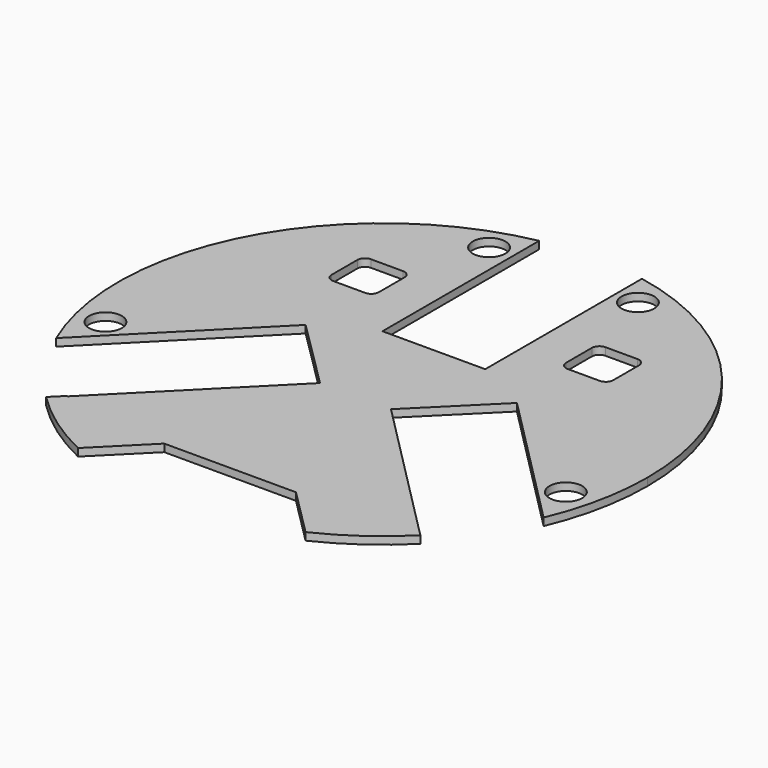
from build123d import *

# Parameters (mm, degrees)
F0_R     = 6.5
F1_DEPTH = 3


with BuildPart() as f1:
    # F0 (on Top) → F1 (new body)
    with BuildSketch(Plane.XY):
        with BuildLine():
            Line((-69.5263431778, -69.5263431778), (-74.2462120246, -74.2462120246))
            ThreePointArc((-74.2462120246, -74.2462120246), (-60.5690845883, -85.7693767736), (-45.1347826829, -94.804279398))
            Line((-45.1347826829, -94.804279398), (-26.1228149757, -75.7923116907))
            Line((-26.1228149757, -75.7923116907), (0, -49.6694967151))
            Line((0, -49.6694967151), (0, 0))
            Line((0, 0), (-13.8767590343, -13.8767590343))
            Line((-13.8767590343, -13.8767590343), (-13.825551364, -13.9276425795))
            Line((-13.825551364, -13.9276425795), (-69.2978968304, -69.7533435465))
            Line((-69.2978968304, -69.7533435465), (-69.5263431778, -69.5263431778))
        make_face()
        Polygon((0, -49.6694967151), (-26.1228149757, -75.7923116907), (0, -75.7923116907), (0, -64.7160249151), align=None)
        with BuildLine():
            ThreePointArc((-20.428937125, 102.9934877939), (-92.9055396428, 48.9240299208), (-96.4815047793, -41.4284833844))
            Line((-96.4815047793, -41.4284833844), (-41.6658031427, 13.7363909711))
            Line((-41.6658031427, 13.7363909711), (-13.8767590343, -13.8767590343))
            Line((-13.8767590343, -13.8767590343), (0, 0))
            Line((0, 0), (0, 25.2874530852))
            Line((0, 25.2874530852), (-20.428937125, 25.2874530852))
            Line((-20.428937125, 25.2874530852), (-20.428937125, 102.9934877939))
        make_face()
        with Locations((-91.3139134645, -23.4654136002)):
            Circle(F0_R, mode=Mode.SUBTRACT)
        with BuildLine():
            ThreePointArc((-56.388001889, 57.7684769799), (-55.5093222326, 59.8897973234), (-53.388001889, 60.7684769799))
            Line((-53.388001889, 60.7684769799), (-40.6683964263, 60.7684769799))
            ThreePointArc((-40.6683964263, 60.7684769799), (-38.5470760828, 59.8897973234), (-37.6683964263, 57.7684769799))
            Line((-37.6683964263, 57.7684769799), (-37.6683964263, 45.0488715172))
            ThreePointArc((-37.6683964263, 45.0488715172), (-38.5470760828, 42.9275511736), (-40.6683964263, 42.0488715172))
            Line((-40.6683964263, 42.0488715172), (-53.388001889, 42.0488715172))
            ThreePointArc((-53.388001889, 42.0488715172), (-55.5093222326, 42.9275511736), (-56.388001889, 45.0488715172))
            Line((-56.388001889, 45.0488715172), (-56.388001889, 57.7684769799))
        make_face(mode=Mode.SUBTRACT)
        with Locations((-29.722429812, 89.7770151496)):
            Circle(F0_R, mode=Mode.SUBTRACT)
        with BuildLine():
            Line((26.1228149757, -75.7923116907), (45.1347826829, -94.804279398))
            ThreePointArc((45.1347826829, -94.804279398), (60.5690845883, -85.7693767736), (74.2462120246, -74.2462120246))
            Line((74.2462120246, -74.2462120246), (69.7533435465, -69.7533435465))
            Line((69.7533435465, -69.7533435465), (0, 0))
            Line((0, 0), (0, -49.6694967151))
            Line((0, -49.6694967151), (26.1228149757, -75.7923116907))
        make_face()
        Polygon((0, -64.7160249151), (0, -75.7923116907), (26.1228149757, -75.7923116907), (0, -49.6694967151), align=None)
        with BuildLine():
            Line((0, 25.2874530852), (0, 0))
            Line((0, 0), (69.7533435465, -69.7533435465))
            Line((69.7533435465, -69.7533435465), (14.3003088274, -13.9084606974))
            Line((14.3003088274, -13.9084606974), (42.1468239183, 13.7426630826))
            Line((42.1468239183, 13.7426630826), (96.6167267267, -41.1121407447))
            ThreePointArc((96.6167267267, -41.1121407447), (102.8828370194, -20.9790811726), (105, 0))
            ThreePointArc((105, 0), (81.1159350321, 66.6723712182), (20.3294269741, 103.013175851))
            Line((20.3294269741, 103.013175851), (20.3294269741, 25.2874530852))
            Line((20.3294269741, 25.2874530852), (0, 25.2874530852))
        make_face()
        with Locations((91.3139144, -23.4654136002)):
            Circle(F0_R, mode=Mode.SUBTRACT)
        with BuildLine():
            ThreePointArc((37.1843986213, 57.0661032964), (38.0630782778, 59.18742364), (40.1843986213, 60.0661032964))
            Line((40.1843986213, 60.0661032964), (52.904004084, 60.0661032964))
            ThreePointArc((52.904004084, 60.0661032964), (55.0253244276, 59.18742364), (55.904004084, 57.0661032964))
            Line((55.904004084, 57.0661032964), (55.904004084, 44.3464978337))
            ThreePointArc((55.904004084, 44.3464978337), (55.0253244276, 42.2251774902), (52.904004084, 41.3464978337))
            Line((52.904004084, 41.3464978337), (40.1843986213, 41.3464978337))
            ThreePointArc((40.1843986213, 41.3464978337), (38.0630782778, 42.2251774902), (37.1843986213, 44.3464978337))
            Line((37.1843986213, 44.3464978337), (37.1843986213, 57.0661032964))
        make_face(mode=Mode.SUBTRACT)
        with Locations((29.2972179146, 89.7770151496)):
            Circle(F0_R, mode=Mode.SUBTRACT)
    extrude(amount=F1_DEPTH)


solid = f1.part
